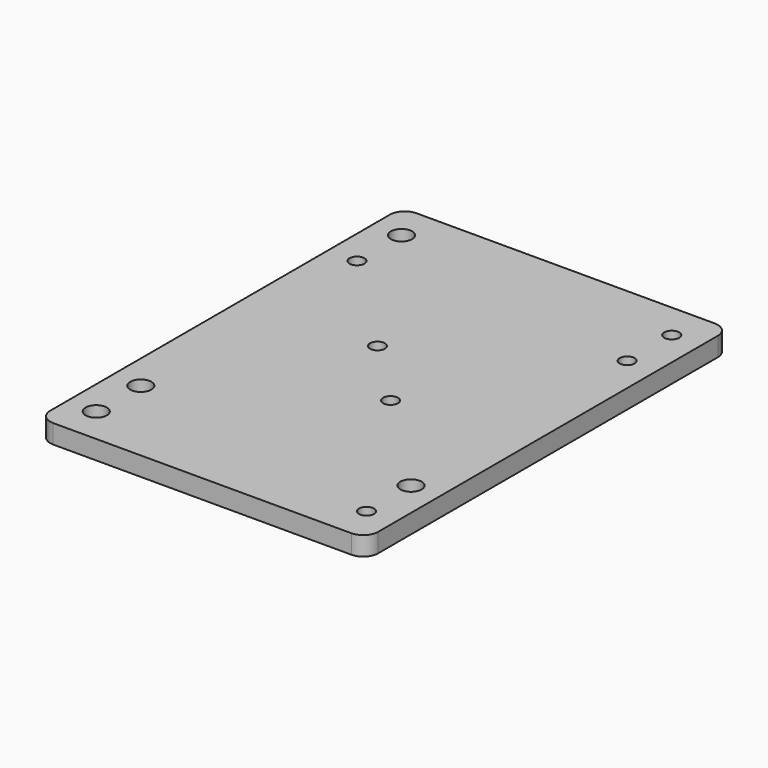
from build123d import *

# Parameters (mm, degrees)
F0_W     = 110
F0_H     = 152.4
F0_R     = 3.56
F0_R_2   = 2.5
F1_DEPTH = 6.35
F2_R     = 5


# Not quite as in the source:
# - a length typed as a fraction of an inch, garbled in the dataset ("3 / 203.2 mm" for 3/8 in), is restored


with BuildPart() as f1:
    # F0 (on Top) → F1 (new body)
    with BuildSketch(Plane.XY):
        Rectangle(F0_W, F0_H)
        with Locations((-45.325, -64)):
            Circle(F0_R, mode=Mode.SUBTRACT)
        with Locations((-45.325, -45.325)):
            Circle(F0_R, mode=Mode.SUBTRACT)
        with Locations((45.325, -64)):
            Circle(F0_R_2, mode=Mode.SUBTRACT)
        with Locations((45.325, -45.325)):
            Circle(F0_R, mode=Mode.SUBTRACT)
        with Locations((11, -11)):
            Circle(F0_R_2, mode=Mode.SUBTRACT)
        with Locations((-11, 11)):
            Circle(F0_R_2, mode=Mode.SUBTRACT)
        with Locations((-45.325, 45.325)):
            Circle(F0_R_2, mode=Mode.SUBTRACT)
        with Locations((-45.325, 64)):
            Circle(F0_R, mode=Mode.SUBTRACT)
        with Locations((45.325, 45.325)):
            Circle(F0_R_2, mode=Mode.SUBTRACT)
        with Locations((45.325, 64)):
            Circle(F0_R_2, mode=Mode.SUBTRACT)
    extrude(amount=F1_DEPTH)

    # F2
    f2_edges = [f1.edges().sort_by_distance(p)[0] for p in [
        (-55, 76.2, 3.175),
        (55, 76.2, 3.175),
        (55, -76.2, 3.175),
        (-55, -76.2, 3.175),
    ]]
    fillet(f2_edges, radius=F2_R)


solid = f1.part
